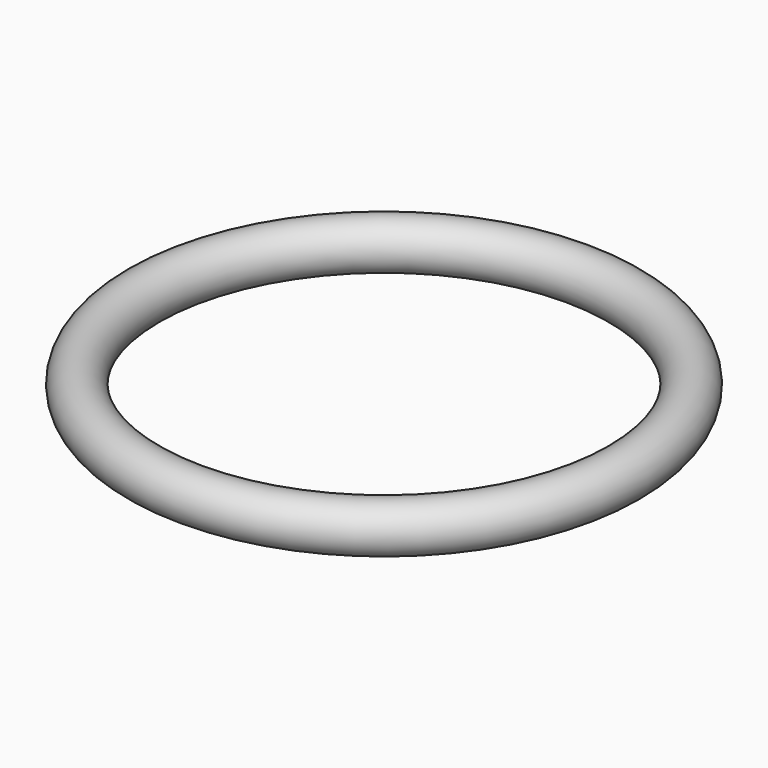
from build123d import *

# Parameters (mm, degrees)
F0_R = 0.5


# Not quite as in the source:
# - a feature names something its author has since deleted; it is built from what else it names


with BuildPart() as f1:
    # F0 (on Front) → F1 (revolve)
    with BuildSketch(Plane.XZ):
        with Locations((-5, 4.0333913639)):
            Circle(F0_R)
    revolve(axis=Axis((0, 0, 33.8092235981), (0, 0, 1)))


solid = f1.part
